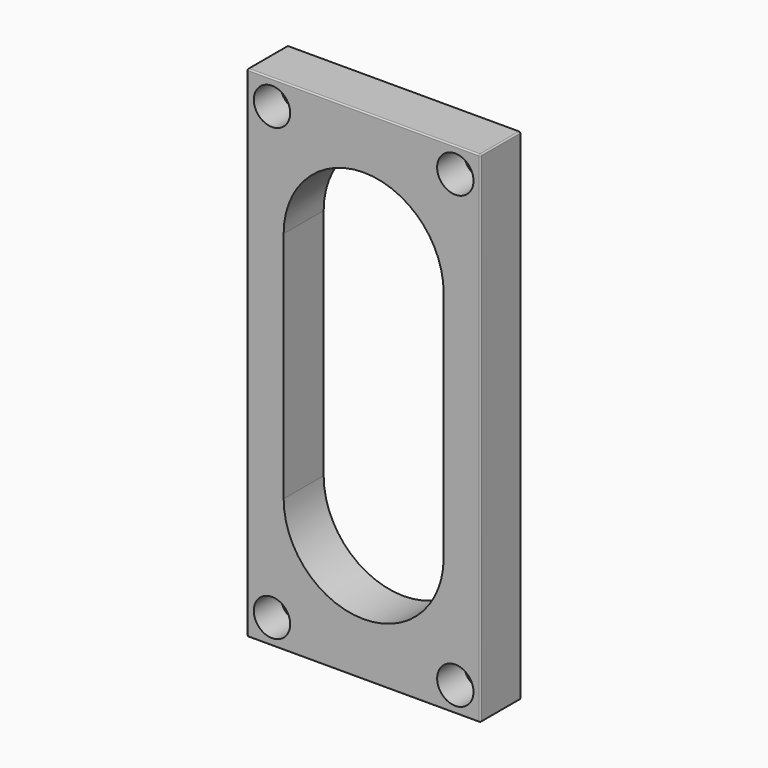
from build123d import *

# Parameters (mm, degrees)
F0_W      = 44.45
F0_H      = 95.25
F0_R      = 3.4671
F1_DEPTH  = 6.35
F0_R_2    = 2.2479
F1_FACE_W = 44.45
F1_FACE_H = 95.25
F1_FACE_R = 3.4671
F2_DEPTH  = 3.175
F3_R      = 0.254


# Not quite as in the source:
# - a feature names something its author has since deleted; it is built from what else it names


with BuildPart() as f1:
    # F0 (on Front) → F1 (new body)
    with BuildSketch(Plane.XZ):
        Rectangle(F0_W, F0_H)
        with Locations((-17.4625, -42.8625)):
            Circle(F0_R, mode=Mode.SUBTRACT)
        with Locations((17.4625, -42.8625)):
            Circle(F0_R, mode=Mode.SUBTRACT)
        with Locations((-17.4625, 42.8625)):
            Circle(F0_R, mode=Mode.SUBTRACT)
        with BuildLine():
            ThreePointArc((-15.24, 22.225), (0, 37.465), (15.24, 22.225))
            Line((15.24, 22.225), (15.24, -22.225))
            ThreePointArc((15.24, -22.225), (0, -37.465), (-15.24, -22.225))
            Line((-15.24, -22.225), (-15.24, 22.225))
        make_face(mode=Mode.SUBTRACT)
        with Locations((17.4625, 42.8625)):
            Circle(F0_R, mode=Mode.SUBTRACT)
    extrude(amount=F1_DEPTH)

    # F0 (on Front) + F1_face (on face) → F2 (join)
    with BuildSketch(Plane.XZ):
        Rectangle(F0_W, F0_H)
        with Locations((-17.4625, -42.8625)):
            Circle(F0_R, mode=Mode.SUBTRACT)
        with Locations((17.4625, -42.8625)):
            Circle(F0_R, mode=Mode.SUBTRACT)
        with Locations((-17.4625, 42.8625)):
            Circle(F0_R, mode=Mode.SUBTRACT)
        with BuildLine():
            ThreePointArc((-15.24, 22.225), (0, 37.465), (15.24, 22.225))
            Line((15.24, 22.225), (15.24, -22.225))
            ThreePointArc((15.24, -22.225), (0, -37.465), (-15.24, -22.225))
            Line((-15.24, -22.225), (-15.24, 22.225))
        make_face(mode=Mode.SUBTRACT)
        with Locations((17.4625, 42.8625)):
            Circle(F0_R, mode=Mode.SUBTRACT)
        with Locations((-17.4625, 42.8625)):
            Circle(F0_R)
        with Locations((-17.4625, 42.8625)):
            Circle(F0_R_2, mode=Mode.SUBTRACT)
        with Locations((17.4625, 42.8625)):
            Circle(F0_R)
        with Locations((17.4625, 42.8625)):
            Circle(F0_R_2, mode=Mode.SUBTRACT)
        with Locations((-17.4625, -42.8625)):
            Circle(F0_R)
        with Locations((-17.4625, -42.8625)):
            Circle(F0_R_2, mode=Mode.SUBTRACT)
        with Locations((17.4625, -42.8625)):
            Circle(F0_R)
        with Locations((17.4625, -42.8625)):
            Circle(F0_R_2, mode=Mode.SUBTRACT)
    with BuildSketch(Plane.XZ.offset(6.35)):
        Rectangle(F1_FACE_W, F1_FACE_H)
        with Locations((-17.4625, -42.8625)):
            Circle(F1_FACE_R, mode=Mode.SUBTRACT)
        with Locations((17.4625, -42.8625)):
            Circle(F1_FACE_R, mode=Mode.SUBTRACT)
        with Locations((-17.4625, 42.8625)):
            Circle(F1_FACE_R, mode=Mode.SUBTRACT)
        with BuildLine():
            Line((-15.24, -22.225), (-15.24, 22.225))
            ThreePointArc((-15.24, 22.225), (0, 37.465), (15.24, 22.225))
            Line((15.24, 22.225), (15.24, -22.225))
            ThreePointArc((15.24, -22.225), (0, -37.465), (-15.24, -22.225))
        make_face(mode=Mode.SUBTRACT)
        with Locations((17.4625, 42.8625)):
            Circle(F1_FACE_R, mode=Mode.SUBTRACT)
    extrude(amount=F2_DEPTH)

    # F3
    f3_edges = [f1.edges().sort_by_distance(p)[0] for p in [
        (-22.225, -9.525, 0),
        (0, -9.525, -47.625),
        (22.225, -9.525, 0),
        (0, -9.525, 47.625),
        (-22.225, -4.7625, 47.625),
        (22.225, -4.7625, 47.625),
        (22.225, -4.7625, -47.625),
        (-22.225, -4.7625, -47.625),
    ]]
    fillet(f3_edges, radius=F3_R)


solid = f1.part
